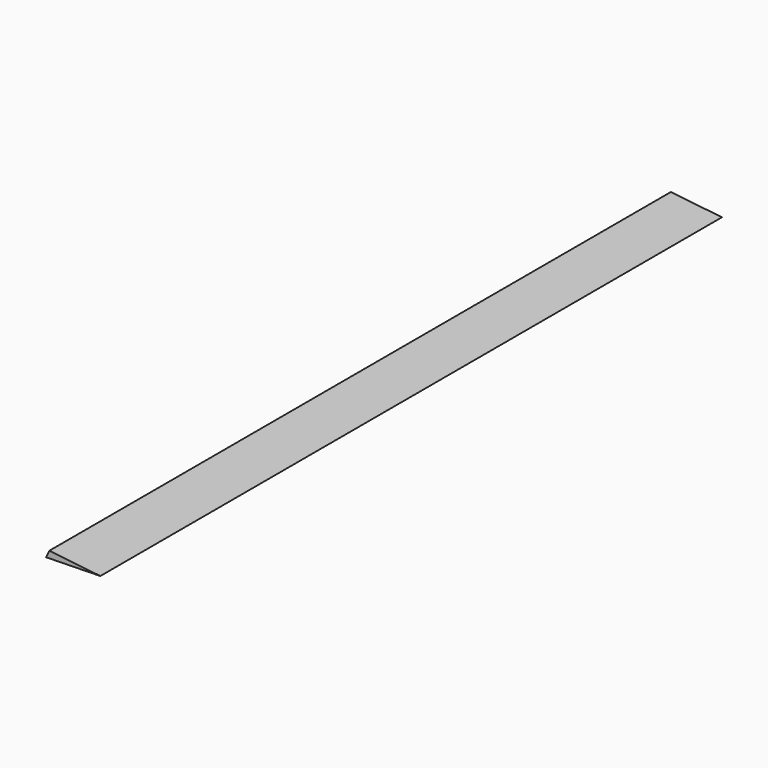
from build123d import *

# Parameters (mm, degrees)
F1_DEPTH = 25.4


with BuildPart() as f1:
    # F0 (on Front) → F1 (new body)
    with BuildSketch(Plane.XZ):
        Polygon((-57.9446703196, -44.5015057921), (-58.0501846598, -44.7235413628), (-56.2758632004, -44.6869283915), align=None)
    extrude(amount=F1_DEPTH)


solid = f1.part
